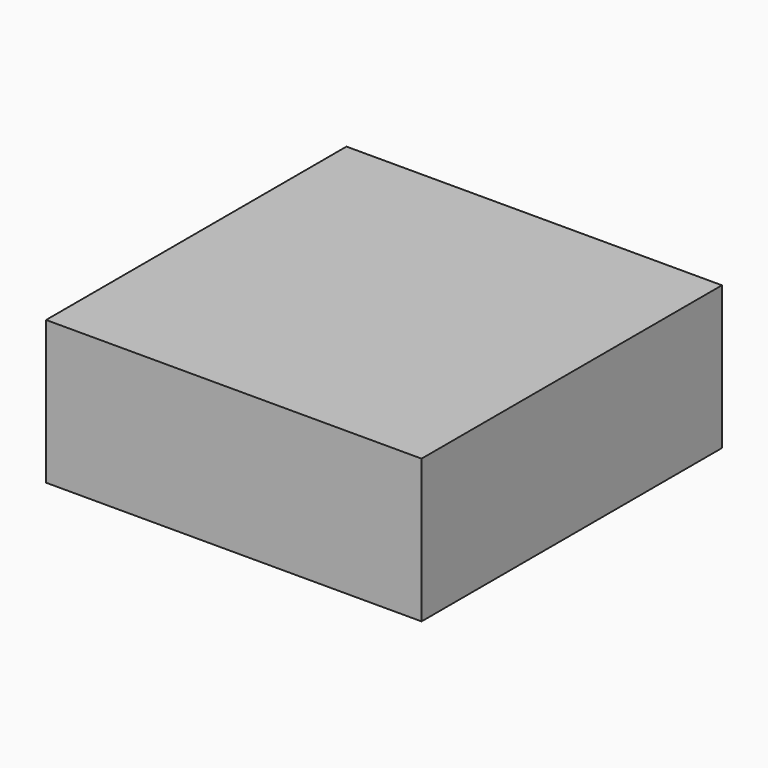
from build123d import *

# Parameters (mm, degrees)
F0_W     = 99.822
F0_H     = 99.822
F1_DEPTH = 38.1


# Not quite as in the source:
# - a feature of the source that left no trace in its solid (it failed there, or was rolled back) is left out


with BuildPart() as f1:
    # F0 (on Top) → F1 (new body)
    with BuildSketch(Plane.XY):
        Rectangle(F0_W, F0_H)
    extrude(amount=F1_DEPTH)


solid = f1.part
